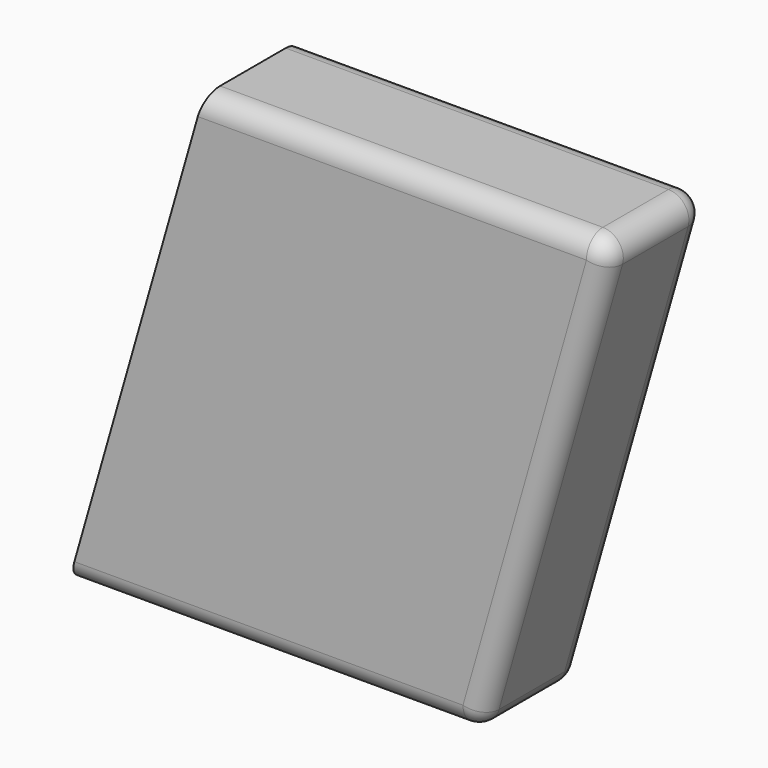
from build123d import *

# Parameters (mm, degrees)
F3_DEPTH = 3.81
F4_R     = 1.27


# Not quite as in the source:
# - the program builds the solid bodies; features that only make, move or delete a surface that nothing else refers to are left out


with BuildPart() as f3:
    # F2 (on Front) → F3 (new body, symmetric)
    with BuildSketch(Plane.XZ):
        Polygon((67.4008423153, 47.9680152879), (42.0008423153, 47.9680152879), (33.6273413479, 18.6607656464), (59.0273413479, 18.6607656464), align=None)
    extrude(amount=F3_DEPTH, both=True)

    # F4
    f4_edges = [f3.edges().sort_by_distance(p)[0] for p in [
        (54.700842, -3.81, 47.968015),
        (63.214092, -3.81, 33.31439),
        (46.327341, -3.81, 18.660766),
        (63.214092, 3.81, 33.31439),
        (54.700842, 3.81, 47.968015),
        (46.327341, 3.81, 18.660766),
        (67.400842, 0, 47.968015),
        (59.027341, 0, 18.660766),
    ]]
    fillet(f4_edges, radius=F4_R)


solid = f3.part
